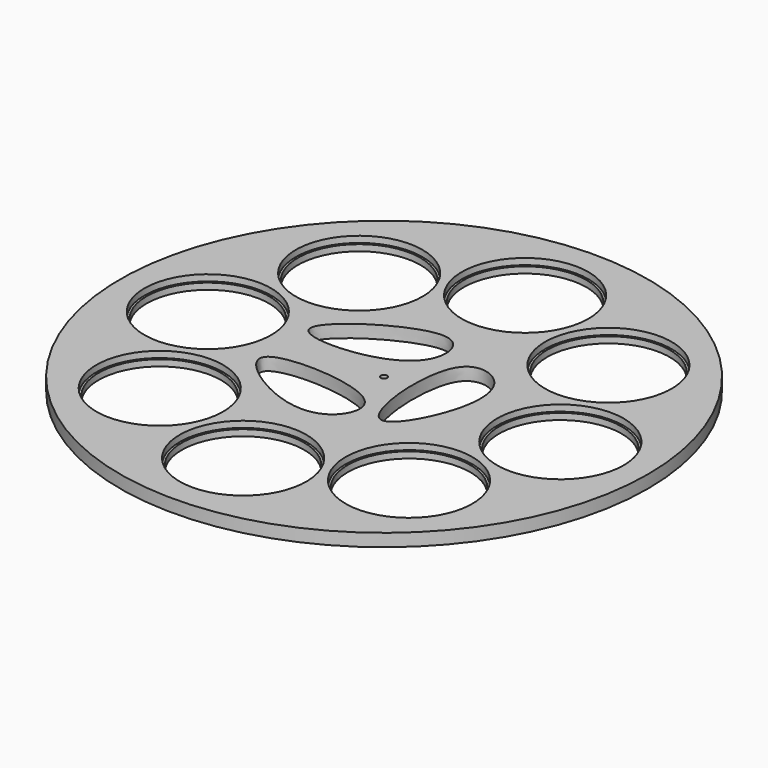
from build123d import *

# Parameters (mm, degrees)
F0_R            = 125
F1_DEPTH        = 3
F2_R            = 1.5
F3_DEPTH        = 6.001
F5_R            = 29
F6_DEPTH        = 6.001
F6_COPIES_COUNT = 8
F5_R_2          = 30
F7_DEPTH        = 3
F7_COPIES_COUNT = 8
F9_DEPTH        = 6.001


# Not quite as in the source:
# - a pattern or mirror of a feature is missing from the dataset's text; its kind, count and spacing are read off the source's solid


with BuildPart() as f1:
    # F0 (on Top) → F1 (new body, symmetric)
    with BuildSketch(Plane.XY):
        Circle(F0_R)
    extrude(amount=F1_DEPTH, both=True)

    # F2 (on face) → F3 (cut, through all)
    with BuildSketch(Plane(origin=(0, 0, -3), x_dir=(1, 0, 0), z_dir=(0, 0, -1))):
        Circle(F2_R)
    extrude(amount=-F3_DEPTH, mode=Mode.SUBTRACT)

    # F5 (on face) → F6 (cut, through all)
    with BuildSketch(Plane.XY.offset(3)):
        with Locations((83.46965909, 0)):
            Circle(F5_R)
    f6 = extrude(amount=-F6_DEPTH, mode=Mode.SUBTRACT)

    # F6_copies: F6 ×8 about axis
    f6_copies_axis = Axis((0, 0, 0), (0, 0, 1))
    for i in range(1, F6_COPIES_COUNT):
        add(f6.rotate(f6_copies_axis, i * 360 / F6_COPIES_COUNT), mode=Mode.SUBTRACT)

    # F5 (on face) → F7 (cut)
    with BuildSketch(Plane.XY.offset(3)):
        with Locations((83.46965909, 0)):
            Circle(F5_R_2)
        with Locations((83.46965909, 0)):
            Circle(F5_R, mode=Mode.SUBTRACT)
    f7 = extrude(amount=-F7_DEPTH, mode=Mode.SUBTRACT)

    # F7_copies: F7 ×8 about axis
    f7_copies_axis = Axis((0, 0, 0), (0, 0, 1))
    for i in range(1, F7_COPIES_COUNT):
        add(f7.rotate(f7_copies_axis, i * 360 / F7_COPIES_COUNT), mode=Mode.SUBTRACT)

    # F8 (on face) → F9 (cut, through all)
    with BuildSketch(Plane.XY.offset(3)):
        with BuildLine():
            add(Edge.make_bspline(
                [(-44.3258620799, -15.0524862111), (-48.3588050122, -20.1152564211), (-23.0924792953, -39.7830257512), (5.512565217, -41.0118510348), (16.0001607542, -11.0681310793), (-38.9619666275, -8.3188997057), (-44.3258620799, -15.0524862111)],
                knots=[0, 0, 0, 0, 0.2444791319, 0.4878585615, 0.6748378229, 1, 1, 1, 1], degree=3))
        make_face()
        with BuildLine():
            add(Edge.make_bspline(
                [(-45.671308504, 13.8018518265), (-46.0710162563, 7.3414722241), (-14.0930848504, 5.7227478351), (10.0436210659, 21.123332585), (1.4595442067, 51.6672296743), (-45.1396891305, 22.3942870163), (-45.671308504, 13.8018518265)],
                knots=[0, 0, 0, 0, 0.2444791319, 0.4878585615, 0.6748378229, 1, 1, 1, 1], degree=3))
        make_face()
        with BuildLine():
            add(Edge.make_bspline(
                [(19.5642778018, -27.1424591751), (25.1230293593, -30.4585641219), (41.2175010078, -2.7786734428), (38.591626534, 25.7320853401), (7.5102643018, 32.1011470227), (12.1710260995, -22.7319727037), (19.5642778018, -27.1424591751)],
                knots=[0, 0, 0, 0, 0.2444791319, 0.4878585615, 0.6748378229, 1, 1, 1, 1], degree=3))
        make_face()
    extrude(amount=-F9_DEPTH, mode=Mode.SUBTRACT)


solid = f1.part
